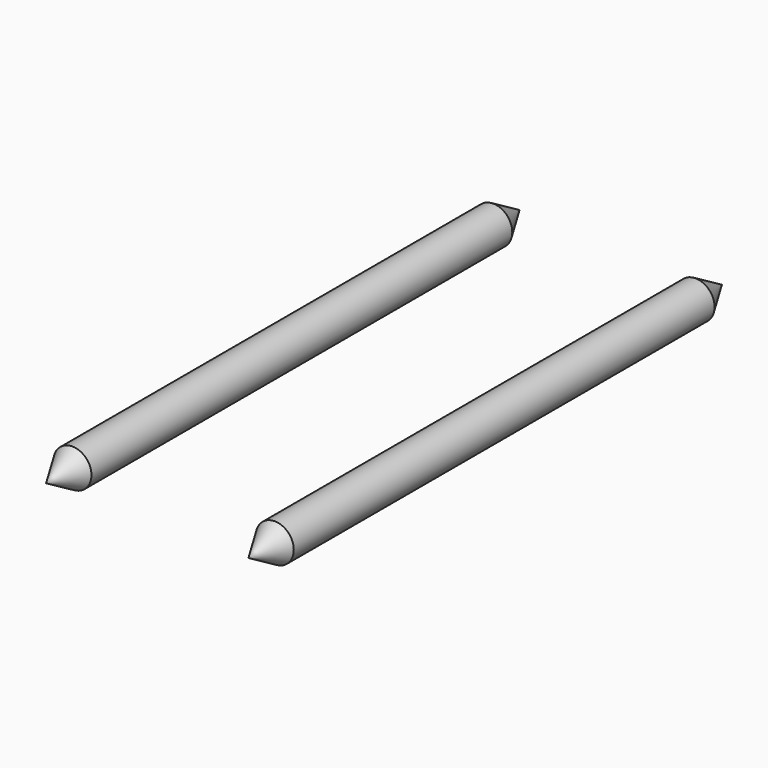
from build123d import *

# Parameters (mm, degrees)
F0_R     = 2.3876
F1_DEPTH = 66.04
F2_R     = 2.3876
F4_R     = 2.3876


# Not quite as in the source:
# - an extrude whose draft closes it to a point is written as a loft to that point


with BuildPart() as f1:
    # F0 (on Front) → F1 (new body)
    with BuildSketch(Plane.XZ):
        Circle(F0_R)
    extrude(amount=F1_DEPTH)

    # F2 (on face) → F3 section 0
    with BuildSketch(Plane.XZ.offset(66.04), mode=Mode.PRIVATE) as f3_s0:
        Circle(F2_R)
    loft([f3_s0.sketch, Vertex(0, -70.1754445082, 0)], ruled=True)

    # F4 (on face) → F5 section 0
    with BuildSketch(Plane(origin=(0, 0, 0), x_dir=(-1, 0, 0), z_dir=(0, 1, 0)), mode=Mode.PRIVATE) as f5_s0:
        Circle(F4_R)
    loft([f5_s0.sketch, Vertex(0, 4.1354445082, 0)], ruled=True)


with BuildPart() as f6_1:
    # F6: copy of F1
    add(f1.part.moved(Location((25.4, 0, 0))))


solid = Compound([f1.part, f6_1.part])
